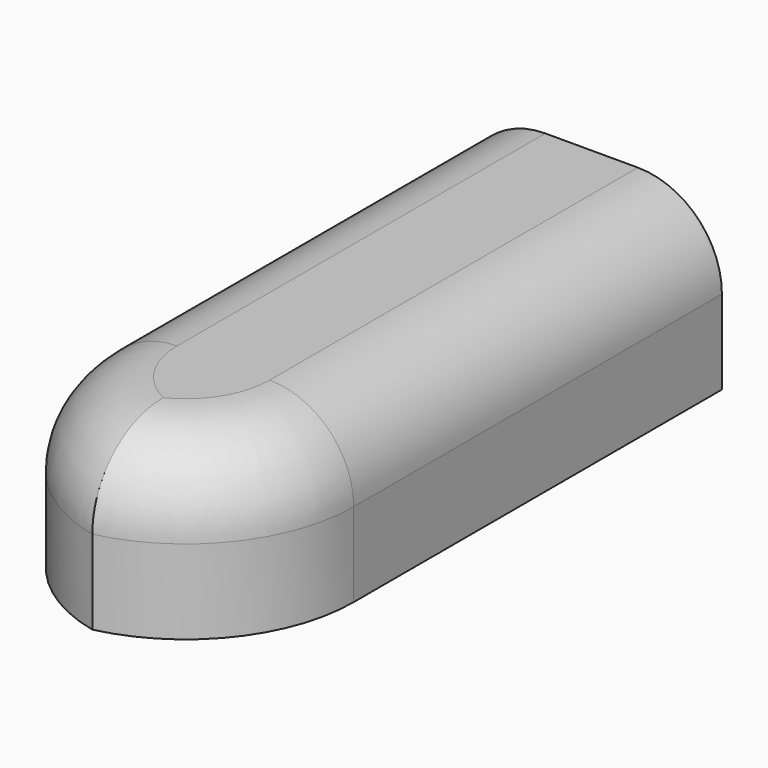
from build123d import *

# Parameters (mm, degrees)
F0_W        = 39.3818542361
F0_H        = 94.9496030807
F1_DEPTH    = 25.4
F2_T1_DEPTH = 152.4
F3_T1_DEPTH = 101.2996030808
F3_T4_ANGLE = 148.6516311692
F3_T6_ANGLE = 148.6516311692


# Not quite as in the source:
# - a fillet or chamfer that OpenCascade refuses, or shapes differently, is made with other operations: its cross-section is extruded or revolved along the edge and cut away or added


with BuildPart() as f1:
    # F0 (on Top) → F1 (new body)
    with BuildSketch(Plane.XY):
        Rectangle(F0_W, F0_H)
    extrude(amount=F1_DEPTH)

    # F2: fillet of radius 25.4 on 2 edges, made by hand

    # F2_s2 → F2_t1 (cut)
    with BuildSketch(Plane.XY.offset(-63.5)):
        with BuildLine():
            ThreePointArc((-5.7090728819, -47.4748015404), (12.2514393602, -40.0353137825), (19.6909271181, -22.0748015404))
            Line((19.6909271181, -22.0748015404), (19.6909271181, -47.4748015404))
            Line((19.6909271181, -47.4748015404), (-5.7090728819, -47.4748015404))
        make_face()
        with BuildLine():
            ThreePointArc((5.7090728819, -47.4748015404), (-12.2514393602, -40.0353137825), (-19.6909271181, -22.0748015404))
            Line((-19.6909271181, -22.0748015404), (-19.6909271181, -47.4748015404))
            Line((-19.6909271181, -47.4748015404), (5.7090728819, -47.4748015404))
        make_face()
    extrude(amount=F2_T1_DEPTH, mode=Mode.SUBTRACT)

    # F3: fillet of radius 12.7 on 4 edges, made by hand

    # F3_s2 → F3_t1 (cut)
    with BuildSketch(Plane.XZ.offset(-79.2248015404)):
        with BuildLine():
            ThreePointArc((6.9909271181, 25.4), (15.9711832391, 21.6802561211), (19.6909271181, 12.7))
            Line((19.6909271181, 12.7), (19.6909271181, 25.4))
            Line((19.6909271181, 25.4), (6.9909271181, 25.4))
        make_face()
        with BuildLine():
            ThreePointArc((-19.6909271181, 12.7), (-15.9711832391, 21.6802561211), (-6.9909271181, 25.4))
            Line((-6.9909271181, 25.4), (-19.6909271181, 25.4))
            Line((-19.6909271181, 25.4), (-19.6909271181, 12.7))
        make_face()
    extrude(amount=F3_T1_DEPTH, mode=Mode.SUBTRACT)

    # F3_s3 → F3_t4 (revolve, cut)
    with BuildSketch(Plane.XZ.offset(22.0748015403)):
        with BuildLine():
            ThreePointArc((6.9909271181, 25.4), (15.9711832392, 21.6802561211), (19.6909271181, 12.7))
            Line((19.6909271181, 12.7), (19.6909271181, 25.4))
            Line((19.6909271181, 25.4), (6.9909271181, 25.4))
        make_face()
    revolve(axis=Axis((-5.709072882, -22.0748015403, 25.4), (0, 0, -1)), revolution_arc=F3_T4_ANGLE, mode=Mode.SUBTRACT)

    # F3_s5 → F3_t6 (revolve, cut)
    with BuildSketch(Plane(origin=(-8.2625761257, -13.5637424397, 0), x_dir=(0, 0, 1), z_dir=(0.5202402568, 0.8540199501, 0))):
        with BuildLine():
            ThreePointArc((12.7, 41.759862561), (21.6802561211, 38.040118682), (25.4, 29.059862561))
            Line((25.4, 29.059862561), (25.4, 41.759862561))
            Line((25.4, 41.759862561), (12.7, 41.759862561))
        make_face()
    revolve(axis=Axis((5.709072882, -22.0748015403, 25.4), (0, 0, -1)), revolution_arc=F3_T6_ANGLE, mode=Mode.SUBTRACT)


solid = f1.part
